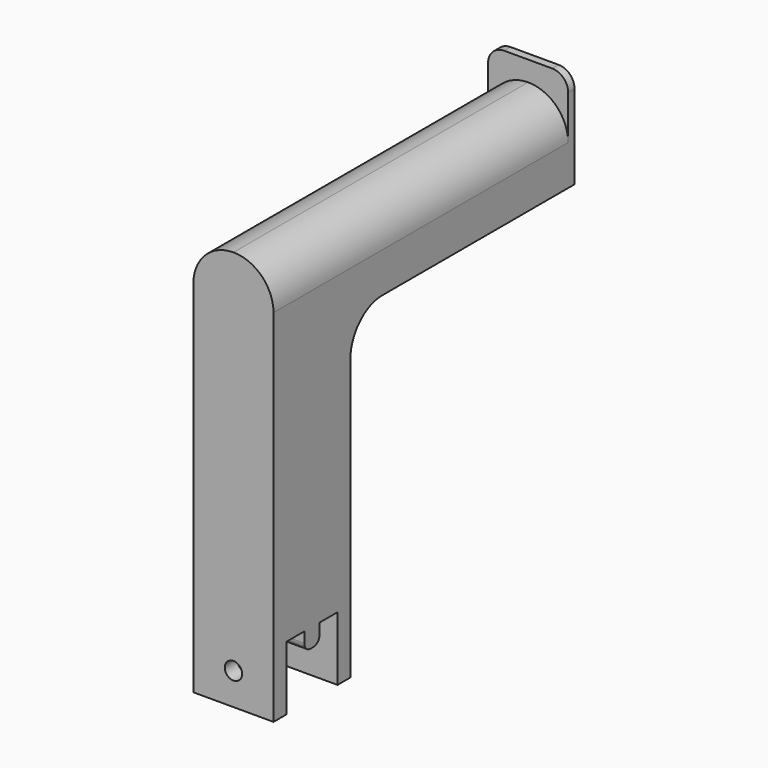
from build123d import *

# Parameters (mm, degrees)
F1_DEPTH = 25.4
F2_R     = 12.69999
F3_R     = 5.08
F4_R     = 12.7
F6_D     = 5.5
F6_DEPTH = 5.588
F6_TIP   = 1.6523667023


# Not quite as in the source:
# - a fillet or chamfer is up to 0.001 mm smaller than in the source, because OpenCascade refuses the exact size


with BuildPart() as f1:
    # F0 (on Right) → F1 (new body)
    with BuildSketch(Plane.YZ):
        with BuildLine():
            Line((3.048, 10.16), (10.16, 10.16))
            Line((10.16, 10.16), (10.16, -10.16))
            Line((10.16, -10.16), (15.24, -10.16))
            Line((15.24, -10.16), (15.24, 91.44))
            Line((15.24, 91.44), (104.14, 91.44))
            Line((104.14, 91.44), (104.14, 123.19))
            Line((104.14, 123.19), (101.6, 123.19))
            Line((101.6, 123.19), (101.6, 116.84))
            Line((101.6, 116.84), (-15.24, 116.84))
            Line((-15.24, 116.84), (-15.24, -10.16))
            Line((-15.24, -10.16), (-10.16, -10.16))
            Line((-10.16, -10.16), (-10.16, 10.16))
            Line((-10.16, 10.16), (-3.048, 10.16))
            Line((-3.048, 10.16), (-3.048, 6.858))
            ThreePointArc((-3.048, 6.858), (-2.3040512242, 5.0619487758), (-0.508, 4.318))
            Line((-0.508, 4.318), (0.508, 4.318))
            ThreePointArc((0.508, 4.318), (2.3040512242, 5.0619487758), (3.048, 6.858))
            Line((3.048, 6.858), (3.048, 10.16))
        make_face()
    extrude(amount=F1_DEPTH)

    # F2 (radius 12.7 in the source; OpenCascade refuses exactly that, so slightly less here)
    f2_edges = [f1.edges().sort_by_distance(p)[0] for p in [
        (25.4, 43.18, 116.84),
        (0, 43.18, 116.84),
    ]]
    fillet(f2_edges, radius=F2_R)

    # F3
    f3_edges = [f1.edges().sort_by_distance(p)[0] for p in [
        (0, 102.87, 123.19),
        (25.4, 102.87, 123.19),
    ]]
    fillet(f3_edges, radius=F3_R)

    # F4
    f4_edges = [f1.edges().sort_by_distance(p)[0] for p in [
        (12.7, 15.24, 91.44),
    ]]
    fillet(f4_edges, radius=F4_R)

    # F6
    with Locations(Plane.XZ.offset(15.24)):
        with Locations((12.7, 0)):
            Hole(F6_D / 2, depth=F6_DEPTH)
            with Locations((0, 0, -(F6_DEPTH + F6_TIP / 2))):  # 118° drill point
                Cone(0, F6_D / 2, F6_TIP, mode=Mode.SUBTRACT)


solid = f1.part
